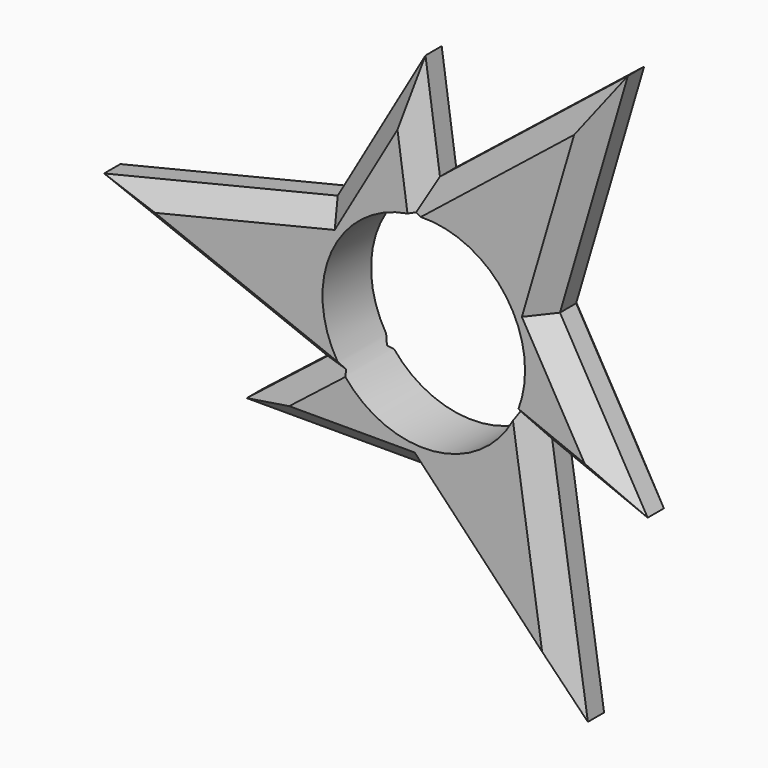
from build123d import *

# Parameters (mm, degrees)
F0_R          = 15
F1_DEPTH      = 9
F2_DEPTH      = 9
F3_T4_DEPTH   = 41.4194656766
F3_T9_DEPTH   = 51.0233182668
F3_T14_DEPTH  = 51.0233182668
F3_T19_DEPTH  = 30.6843352159
F3_T24_DEPTH  = 41.4194656766
F3_T29_DEPTH  = 51.0233182668
F3_T34_DEPTH  = 51.0233182668
F3_T39_DEPTH  = 30.6843352159
F3_T44_DEPTH  = 41.4194656766
F3_T49_DEPTH  = 51.0233182668
F3_T54_DEPTH  = 51.0233182668
F3_T59_DEPTH  = 30.6843352159
F3_T64_DEPTH  = 51.0233182668
F3_T69_DEPTH  = 41.4194656766
F3_T74_DEPTH  = 51.0233182668
F3_T79_DEPTH  = 51.0233182668
F3_T84_DEPTH  = 41.4194656766
F3_T89_DEPTH  = 30.6843352159
F3_T94_DEPTH  = 51.0233182668
F3_T99_DEPTH  = 51.0233182668
F3_T104_DEPTH = 41.4194656766
F3_T109_DEPTH = 51.0233182668
F3_T114_DEPTH = 30.6843352159
F3_T119_DEPTH = 30.6843352159
F3_T125_DEPTH = 51.0233182668
F3_T129_DEPTH = 41.4194656766
F3_T136_DEPTH = 51.0233182668
F3_T140_DEPTH = 30.6843352159
F3_T147_DEPTH = 41.4194656766
F3_T151_DEPTH = 51.0233182668
F3_T158_DEPTH = 51.0233182668
F3_T162_DEPTH = 30.6843352159
F3_T169_DEPTH = 41.4194656766
F3_T173_DEPTH = 51.0233182668
F3_T180_DEPTH = 51.0233182668
F3_T184_DEPTH = 30.6843352159
F3_T191_DEPTH = 41.4194656766
F3_T195_DEPTH = 51.0233182668
F3_T202_DEPTH = 51.0233182668
F3_T206_DEPTH = 30.6843352159
F3_T213_DEPTH = 41.4194656766
F3_T217_DEPTH = 51.0233182668
F3_T224_DEPTH = 51.0233182668
F3_T228_DEPTH = 30.6843352159
F3_T235_DEPTH = 51.0233182668
F3_T239_DEPTH = 41.4194656766
F3_T246_DEPTH = 51.0233182668
F3_T250_DEPTH = 30.6843352159


# Not quite as in the source:
# - a fillet or chamfer that OpenCascade refuses, or shapes differently, is made with other operations: its cross-section is extruded or revolved along the edge and cut away or added


with BuildPart() as f1:
    # F0 (on Front) → F1 (new body)
    with BuildSketch(Plane.XZ):
        with BuildLine():
            ThreePointArc((-16.6111198958, -9.5904345434), (-19.1355906319, 1.3171598584), (-15.1404052923, 11.7759868593))
            Line((-15.1404052923, 11.7759868593), (-49.7397878859, 3.4237381657))
            Line((-49.7397878859, 3.4237381657), (-16.6111198958, -9.5904345434))
        make_face()
        with BuildLine():
            ThreePointArc((0, 19.1808690868), (10.7084892142, 15.9133276745), (17.7685064209, 7.2239821771))
            Line((17.7685064209, 7.2239821771), (27.8349381703, 41.3640508052))
            Line((27.8349381703, 41.3640508052), (0, 19.1808690868))
        make_face()
        with BuildLine():
            Line((21.9048497156, -44.7877889709), (16.6111198958, -9.5904345434))
            ThreePointArc((16.6111198958, -9.5904345434), (8.4271014177, -17.2304875329), (-2.6281011286, -18.9999690364))
            Line((-2.6281011286, -18.9999690364), (21.9048497156, -44.7877889709))
        make_face()
        with BuildLine():
            ThreePointArc((16.6111198958, -9.5904345434), (18.5272968216, -4.9643742213), (19.1808690868, 0))
            ThreePointArc((19.1808690868, 0), (18.8244672495, 3.6803765702), (17.7685064209, 7.2239821771))
            ThreePointArc((17.7685064209, 7.2239821771), (10.7084892142, 15.9133276745), (0, 19.1808690868))
            ThreePointArc((0, 19.1808690868), (-8.4271014177, 17.2304875329), (-15.1404052923, 11.7759868593))
            ThreePointArc((-15.1404052923, 11.7759868593), (-19.1355906319, 1.3171598584), (-16.6111198958, -9.5904345434))
            ThreePointArc((-16.6111198958, -9.5904345434), (-10.7084892142, -15.9133276745), (-2.6281011286, -18.9999690364))
            ThreePointArc((-2.6281011286, -18.9999690364), (8.4271014177, -17.2304875329), (16.6111198958, -9.5904345434))
        make_face()
        Circle(F0_R, mode=Mode.SUBTRACT)
    extrude(amount=F1_DEPTH)

    # F0 (on Front) → F2 (join)
    with BuildSketch(Plane.XZ):
        with BuildLine():
            ThreePointArc((16.6111198958, -9.5904345434), (18.5272968216, -4.9643742213), (19.1808690868, 0))
            ThreePointArc((19.1808690868, 0), (18.8244672495, 3.6803765702), (17.7685064209, 7.2239821771))
            ThreePointArc((17.7685064209, 7.2239821771), (10.7084892142, 15.9133276745), (0, 19.1808690868))
            ThreePointArc((0, 19.1808690868), (-8.4271014177, 17.2304875329), (-15.1404052923, 11.7759868593))
            ThreePointArc((-15.1404052923, 11.7759868593), (-19.1355906319, 1.3171598584), (-16.6111198958, -9.5904345434))
            ThreePointArc((-16.6111198958, -9.5904345434), (-10.7084892142, -15.9133276745), (-2.6281011286, -18.9999690364))
            ThreePointArc((-2.6281011286, -18.9999690364), (8.4271014177, -17.2304875329), (16.6111198958, -9.5904345434))
        make_face()
        Circle(F0_R, mode=Mode.SUBTRACT)
        with BuildLine():
            ThreePointArc((17.7685064209, 7.2239821771), (18.8244672495, 3.6803765702), (19.1808690868, 0))
            ThreePointArc((19.1808690868, 0), (18.5272968216, -4.9643742213), (16.6111198958, -9.5904345434))
            Line((16.6111198958, -9.5904345434), (30.7631902953, -15.2834705217))
            Line((30.7631902953, -15.2834705217), (17.7685064209, 7.2239821771))
        make_face()
        with BuildLine():
            ThreePointArc((0, 19.1808690868), (10.7084892142, 15.9133276745), (17.7685064209, 7.2239821771))
            Line((17.7685064209, 7.2239821771), (27.8349381703, 41.3640508052))
            Line((27.8349381703, 41.3640508052), (0, 19.1808690868))
        make_face()
        with BuildLine():
            Line((21.9048497156, -44.7877889709), (16.6111198958, -9.5904345434))
            ThreePointArc((16.6111198958, -9.5904345434), (8.4271014177, -17.2304875329), (-2.6281011286, -18.9999690364))
            Line((-2.6281011286, -18.9999690364), (21.9048497156, -44.7877889709))
        make_face()
        with BuildLine():
            ThreePointArc((-15.1404052923, 11.7759868593), (-8.4271014177, 17.2304875329), (0, 19.1808690868))
            Line((0, 19.1808690868), (-2.1457214179, 34.2834395581))
            Line((-2.1457214179, 34.2834395581), (-15.1404052923, 11.7759868593))
        make_face()
        with BuildLine():
            Line((-28.6174688775, -18.9999690364), (-2.6281011286, -18.9999690364))
            ThreePointArc((-2.6281011286, -18.9999690364), (-10.7084892142, -15.9133276745), (-16.6111198958, -9.5904345434))
            Line((-16.6111198958, -9.5904345434), (-28.6174688775, -18.9999690364))
        make_face()
        with BuildLine():
            ThreePointArc((-16.6111198958, -9.5904345434), (-19.1355906319, 1.3171598584), (-15.1404052923, 11.7759868593))
            Line((-15.1404052923, 11.7759868593), (-49.7397878859, 3.4237381657))
            Line((-49.7397878859, 3.4237381657), (-16.6111198958, -9.5904345434))
        make_face()
    extrude(amount=F2_DEPTH)

    # F3: chamfer of 3 on 24 edges, made by hand


with BuildPart() as f3_tool2:
    # F3_s3 → F3_t4 (new body)
    with BuildSketch(Plane(origin=(18.1662589207, 0, 31.4648834341), x_dir=(0, 1, 0), z_dir=(-0.5, 0, -0.8660254038))):
        Polygon((-6, -18.9999690364), (-9, -15.9999690364), (-9, -18.9999690364), align=None)
    extrude(amount=F3_T4_DEPTH)

    split(bisect_by=Plane(origin=(-3.5198762352, 0, 14.5811683787), x_dir=(0, 1, 0), z_dir=(-0.2346584157, 0, 0.9720778919)), keep=Keep.TOP)


with BuildPart() as f1_1:
    add(f1.part)

    # F3_t1: cut F3_tool2
    add(f3_tool2.part, mode=Mode.SUBTRACT)


with BuildPart() as f3_tool7:
    # F3_s8 → F3_t9 (new body)
    with BuildSketch(Plane(origin=(-4.1209005243, 0, -0.9947803527), x_dir=(0, 1, 0), z_dir=(-0.9720778919, 0, -0.2346584157))):
        Polygon((-6, -15), (-9, -12), (-9, -15), align=None)
    extrude(amount=F3_T9_DEPTH)

    split(bisect_by=Plane(origin=(-16.4544558566, 0, 9.4999845182), x_dir=(0, 1, 0), z_dir=(-0.8660254038, 0, 0.5)), keep=Keep.TOP)


with BuildPart() as f1_2:
    add(f1_1.part)

    # F3_t6: cut F3_tool7
    add(f3_tool7.part, mode=Mode.SUBTRACT)


with BuildPart() as f3_tool12:
    # F3_s13 → F3_t14 (new body)
    with BuildSketch(Plane(origin=(-51.4360857888, 0, 20.2060072), x_dir=(0, 1, 0), z_dir=(0.930757815, 0, -0.3656362809))):
        Polygon((-6, -15), (-9, -12), (-9, -15), align=None)
    extrude(amount=F3_T14_DEPTH)

    split(bisect_by=Plane(origin=(-1.6642890677, 0, 2.1235944635), x_dir=(0, 1, 0), z_dir=(-0.6168472612, 0, 0.7870828777)), keep=Keep.TOP)


with BuildPart() as f1_3:
    add(f1_2.part)

    # F3_t11: cut F3_tool12
    add(f3_tool12.part, mode=Mode.SUBTRACT)


with BuildPart() as f3_tool17:
    # F3_s18 → F3_t19 (new body)
    with BuildSketch(Plane(origin=(-8.8744478881, 0, -6.9550221835), x_dir=(0, 1, 0), z_dir=(-0.7870828777, 0, -0.6168472612))):
        Polygon((-9, 0.3019430054), (-6, -2.6980569946), (-9, -2.6980569946), align=None)
    extrude(amount=F3_T19_DEPTH)

    split(bisect_by=Plane(origin=(-5.4845442131, 0, -13.9613672244), x_dir=(0, 1, 0), z_dir=(-0.3656362809, 0, -0.930757815)), keep=Keep.TOP)


with BuildPart() as f1_4:
    add(f1_3.part)

    # F3_t16: cut F3_tool17
    add(f3_tool17.part, mode=Mode.SUBTRACT)


with BuildPart() as f3_tool22:
    # F3_s23 → F3_t24 (new body)
    with BuildSketch(Plane.YZ.offset(-36.3325178414)):
        Polygon((-9, -15.9999690364), (-6, -18.9999690364), (-9, -18.9999690364), align=None)
    extrude(amount=F3_T24_DEPTH)

    split(bisect_by=Plane(origin=(-10.8677241153, 0, -10.3388864272), x_dir=(0, 1, 0), z_dir=(-0.724514941, 0, -0.6892590951)), keep=Keep.TOP)


with BuildPart() as f1_5:
    add(f1_4.part)

    # F3_t21: cut F3_tool22
    add(f3_tool22.part, mode=Mode.SUBTRACT)


with BuildPart() as f3_tool27:
    # F3_s28 → F3_t29 (new body)
    with BuildSketch(Plane(origin=(2.9219553188, 0, -3.0714143641), x_dir=(0, 1, 0), z_dir=(0.6892590951, 0, -0.724514941))):
        Polygon((-9, -12), (-6, -15), (-9, -15), align=None)
    extrude(amount=F3_T29_DEPTH)

    split(bisect_by=Plane.XY.offset(-18.9999690364), keep=Keep.BOTTOM)


with BuildPart() as f1_6:
    add(f1_5.part)

    # F3_t26: cut F3_tool27
    add(f3_tool27.part, mode=Mode.SUBTRACT)


with BuildPart() as f3_tool32:
    # F3_s33 → F3_t34 (new body)
    with BuildSketch(Plane(origin=(8.2191273501, 0, -54.6479605643), x_dir=(0, 1, 0), z_dir=(-0.1487285997, 0, 0.988878053))):
        Polygon((-9, -12), (-6, -15), (-9, -15), align=None)
    extrude(amount=F3_T34_DEPTH)

    split(bisect_by=Plane(origin=(-1.0069422189, 0, -2.5031138436), x_dir=(0, 1, 0), z_dir=(-0.3732101364, 0, -0.9277468373)), keep=Keep.TOP)


with BuildPart() as f1_7:
    add(f1_6.part)

    # F3_t31: cut F3_tool32
    add(f3_tool32.part, mode=Mode.SUBTRACT)


with BuildPart() as f3_tool37:
    # F3_s38 → F3_t39 (new body)
    with BuildSketch(Plane(origin=(10.4604498388, 0, -4.207986224), x_dir=(0, 1, 0), z_dir=(0.9277468373, 0, -0.3732101364))):
        Polygon((-9, 0.3019430054), (-6, -2.6980569946), (-9, -2.6980569946), align=None)
    extrude(amount=F3_T39_DEPTH)

    split(bisect_by=Plane(origin=(14.8331707944, 0, 2.2309289955), x_dir=(0, 1, 0), z_dir=(0.988878053, 0, 0.1487285997)), keep=Keep.TOP)


with BuildPart() as f1_8:
    add(f1_7.part)

    # F3_t36: cut F3_tool37
    add(f3_tool37.part, mode=Mode.SUBTRACT)


with BuildPart() as f3_tool42:
    # F3_s43 → F3_t44 (new body)
    with BuildSketch(Plane(origin=(18.1662589207, 0, -31.4648834341), x_dir=(0, 1, 0), z_dir=(-0.5, 0, 0.8660254038))):
        Polygon((-9, -15.9999690364), (-6, -18.9999690364), (-9, -18.9999690364), align=None)
    extrude(amount=F3_T44_DEPTH)

    split(bisect_by=Plane(origin=(14.3876003504, 0, -4.2422819515), x_dir=(0, 1, 0), z_dir=(0.9591733567, 0, -0.2828187968)), keep=Keep.TOP)


with BuildPart() as f1_9:
    add(f1_8.part)

    # F3_t41: cut F3_tool42
    add(f3_tool42.part, mode=Mode.SUBTRACT)


with BuildPart() as f3_tool47:
    # F3_s48 → F3_t49 (new body)
    with BuildSketch(Plane(origin=(1.1989452055, 0, 4.0661947169), x_dir=(0, 1, 0), z_dir=(0.2828187968, 0, 0.9591733567))):
        Polygon((-9, -12), (-6, -15), (-9, -15), align=None)
    extrude(amount=F3_T49_DEPTH)

    split(bisect_by=Plane(origin=(16.4544558566, 0, 9.4999845182), x_dir=(0, 1, 0), z_dir=(0.8660254038, 0, 0.5)), keep=Keep.TOP)


with BuildPart() as f1_10:
    add(f1_9.part)

    # F3_t46: cut F3_tool47
    add(f3_tool47.part, mode=Mode.SUBTRACT)


with BuildPart() as f3_tool52:
    # F3_s53 → F3_t54 (new body)
    with BuildSketch(Plane(origin=(43.2169584386, 0, 34.4419533643), x_dir=(0, 1, 0), z_dir=(-0.7820292153, 0, -0.6232417721))):
        Polygon((-9, -12), (-6, -15), (-9, -15), align=None)
    extrude(amount=F3_T54_DEPTH)

    split(bisect_by=Plane(origin=(2.6712312866, 0, 0.3795193801), x_dir=(0, 1, 0), z_dir=(0.9900573976, 0, 0.1406639596)), keep=Keep.TOP)


with BuildPart() as f1_11:
    add(f1_10.part)

    # F3_t51: cut F3_tool52
    add(f3_tool52.part, mode=Mode.SUBTRACT)


with BuildPart() as f3_tool57:
    # F3_s58 → F3_t59 (new body)
    with BuildSketch(Plane(origin=(-1.5860019507, 0, 11.1630084074), x_dir=(0, 1, 0), z_dir=(-0.1406639596, 0, 0.9900573976))):
        Polygon((-9, 0.3019430054), (-6, -2.6980569946), (-9, -2.6980569946), align=None)
    extrude(amount=F3_T59_DEPTH)

    split(bisect_by=Plane(origin=(-9.3486265813, 0, 11.7304382289), x_dir=(0, 1, 0), z_dir=(-0.6232417721, 0, 0.7820292153)), keep=Keep.TOP)


with BuildPart() as f1_12:
    add(f1_11.part)

    # F3_t56: cut F3_tool57
    add(f3_tool57.part, mode=Mode.SUBTRACT)


with BuildPart() as f3_tool62:
    # F3_s63 → F3_t64 (new body)
    with BuildSketch(Plane(origin=(1.1989452055, 0, 4.0661947169), x_dir=(0, 1, 0), z_dir=(0.2828187968, 0, 0.9591733567))):
        Polygon((0, -12), (-3, -15), (0, -15), align=None)
    extrude(amount=F3_T64_DEPTH)

    split(bisect_by=Plane(origin=(16.4544558566, 0, 9.4999845182), x_dir=(0, 1, 0), z_dir=(0.8660254038, 0, 0.5)), keep=Keep.TOP)


with BuildPart() as f1_13:
    add(f1_12.part)

    # F3_t61: cut F3_tool62
    add(f3_tool62.part, mode=Mode.SUBTRACT)


with BuildPart() as f3_tool67:
    # F3_s68 → F3_t69 (new body)
    with BuildSketch(Plane(origin=(18.1662589207, 0, -31.4648834341), x_dir=(0, 1, 0), z_dir=(-0.5, 0, 0.8660254038))):
        Polygon((0, -15.9999690364), (-3, -18.9999690364), (0, -18.9999690364), align=None)
    extrude(amount=F3_T69_DEPTH)

    split(bisect_by=Plane(origin=(14.3876003504, 0, -4.2422819515), x_dir=(0, 1, 0), z_dir=(0.9591733567, 0, -0.2828187968)), keep=Keep.TOP)


with BuildPart() as f1_14:
    add(f1_13.part)

    # F3_t66: cut F3_tool67
    add(f3_tool67.part, mode=Mode.SUBTRACT)


with BuildPart() as f3_tool72:
    # F3_s73 → F3_t74 (new body)
    with BuildSketch(Plane(origin=(8.2191273501, 0, -54.6479605643), x_dir=(0, 1, 0), z_dir=(-0.1487285997, 0, 0.988878053))):
        Polygon((0, -12), (-3, -15), (0, -15), align=None)
    extrude(amount=F3_T74_DEPTH)

    split(bisect_by=Plane(origin=(-1.0069422189, 0, -2.5031138436), x_dir=(0, 1, 0), z_dir=(-0.3732101364, 0, -0.9277468373)), keep=Keep.TOP)


with BuildPart() as f1_15:
    add(f1_14.part)

    # F3_t71: cut F3_tool72
    add(f3_tool72.part, mode=Mode.SUBTRACT)


with BuildPart() as f3_tool77:
    # F3_s78 → F3_t79 (new body)
    with BuildSketch(Plane(origin=(2.9219553188, 0, -3.0714143641), x_dir=(0, 1, 0), z_dir=(0.6892590951, 0, -0.724514941))):
        Polygon((0, -12), (-3, -15), (0, -15), align=None)
    extrude(amount=F3_T79_DEPTH)

    split(bisect_by=Plane.XY.offset(-18.9999690364), keep=Keep.BOTTOM)


with BuildPart() as f1_16:
    add(f1_15.part)

    # F3_t76: cut F3_tool77
    add(f3_tool77.part, mode=Mode.SUBTRACT)


with BuildPart() as f3_tool82:
    # F3_s83 → F3_t84 (new body)
    with BuildSketch(Plane.YZ.offset(-36.3325178414)):
        Polygon((0, -15.9999690364), (-3, -18.9999690364), (0, -18.9999690364), align=None)
    extrude(amount=F3_T84_DEPTH)

    split(bisect_by=Plane(origin=(-10.8677241153, 0, -10.3388864272), x_dir=(0, 1, 0), z_dir=(-0.724514941, 0, -0.6892590951)), keep=Keep.TOP)


with BuildPart() as f1_17:
    add(f1_16.part)

    # F3_t81: cut F3_tool82
    add(f3_tool82.part, mode=Mode.SUBTRACT)


with BuildPart() as f3_tool87:
    # F3_s88 → F3_t89 (new body)
    with BuildSketch(Plane(origin=(-8.8744478881, 0, -6.9550221835), x_dir=(0, 1, 0), z_dir=(-0.7870828777, 0, -0.6168472612))):
        Polygon((0, 0.3019430054), (-3, -2.6980569946), (0, -2.6980569946), align=None)
    extrude(amount=F3_T89_DEPTH)

    split(bisect_by=Plane(origin=(-5.4845442131, 0, -13.9613672244), x_dir=(0, 1, 0), z_dir=(-0.3656362809, 0, -0.930757815)), keep=Keep.TOP)


with BuildPart() as f1_18:
    add(f1_17.part)

    # F3_t86: cut F3_tool87
    add(f3_tool87.part, mode=Mode.SUBTRACT)


with BuildPart() as f3_tool92:
    # F3_s93 → F3_t94 (new body)
    with BuildSketch(Plane(origin=(-51.4360857888, 0, 20.2060072), x_dir=(0, 1, 0), z_dir=(0.930757815, 0, -0.3656362809))):
        Polygon((-3, -15), (0, -12), (0, -15), align=None)
    extrude(amount=F3_T94_DEPTH)

    split(bisect_by=Plane(origin=(-1.6642890677, 0, 2.1235944635), x_dir=(0, 1, 0), z_dir=(-0.6168472612, 0, 0.7870828777)), keep=Keep.TOP)


with BuildPart() as f1_19:
    add(f1_18.part)

    # F3_t91: cut F3_tool92
    add(f3_tool92.part, mode=Mode.SUBTRACT)


with BuildPart() as f3_tool97:
    # F3_s98 → F3_t99 (new body)
    with BuildSketch(Plane(origin=(-4.1209005243, 0, -0.9947803527), x_dir=(0, 1, 0), z_dir=(-0.9720778919, 0, -0.2346584157))):
        Polygon((-3, -15), (0, -12), (0, -15), align=None)
    extrude(amount=F3_T99_DEPTH)

    split(bisect_by=Plane(origin=(-16.4544558566, 0, 9.4999845182), x_dir=(0, 1, 0), z_dir=(-0.8660254038, 0, 0.5)), keep=Keep.TOP)


with BuildPart() as f1_20:
    add(f1_19.part)

    # F3_t96: cut F3_tool97
    add(f3_tool97.part, mode=Mode.SUBTRACT)


with BuildPart() as f3_tool102:
    # F3_s103 → F3_t104 (new body)
    with BuildSketch(Plane(origin=(18.1662589207, 0, 31.4648834341), x_dir=(0, 1, 0), z_dir=(-0.5, 0, -0.8660254038))):
        Polygon((-3, -18.9999690364), (0, -15.9999690364), (0, -18.9999690364), align=None)
    extrude(amount=F3_T104_DEPTH)

    split(bisect_by=Plane(origin=(-3.5198762352, 0, 14.5811683787), x_dir=(0, 1, 0), z_dir=(-0.2346584157, 0, 0.9720778919)), keep=Keep.TOP)


with BuildPart() as f1_21:
    add(f1_20.part)

    # F3_t101: cut F3_tool102
    add(f3_tool102.part, mode=Mode.SUBTRACT)


with BuildPart() as f3_tool107:
    # F3_s108 → F3_t109 (new body)
    with BuildSketch(Plane(origin=(43.2169584386, 0, 34.4419533643), x_dir=(0, 1, 0), z_dir=(-0.7820292153, 0, -0.6232417721))):
        Polygon((0, -12), (-3, -15), (0, -15), align=None)
    extrude(amount=F3_T109_DEPTH)

    split(bisect_by=Plane(origin=(2.6712312866, 0, 0.3795193801), x_dir=(0, 1, 0), z_dir=(0.9900573976, 0, 0.1406639596)), keep=Keep.TOP)


with BuildPart() as f1_22:
    add(f1_21.part)

    # F3_t106: cut F3_tool107
    add(f3_tool107.part, mode=Mode.SUBTRACT)


with BuildPart() as f3_tool112:
    # F3_s113 → F3_t114 (new body)
    with BuildSketch(Plane(origin=(10.4604498388, 0, -4.207986224), x_dir=(0, 1, 0), z_dir=(0.9277468373, 0, -0.3732101364))):
        Polygon((0, 0.3019430054), (-3, -2.6980569946), (0, -2.6980569946), align=None)
    extrude(amount=F3_T114_DEPTH)

    split(bisect_by=Plane(origin=(14.8331707944, 0, 2.2309289955), x_dir=(0, 1, 0), z_dir=(0.988878053, 0, 0.1487285997)), keep=Keep.TOP)


with BuildPart() as f1_23:
    add(f1_22.part)

    # F3_t111: cut F3_tool112
    add(f3_tool112.part, mode=Mode.SUBTRACT)


with BuildPart() as f3_tool117:
    # F3_s118 → F3_t119 (new body)
    with BuildSketch(Plane(origin=(-1.5860019507, 0, 11.1630084074), x_dir=(0, 1, 0), z_dir=(-0.1406639596, 0, 0.9900573976))):
        Polygon((0, 0.3019430054), (-3, -2.6980569946), (0, -2.6980569946), align=None)
    extrude(amount=F3_T119_DEPTH)

    split(bisect_by=Plane(origin=(-9.3486265813, 0, 11.7304382289), x_dir=(0, 1, 0), z_dir=(-0.6232417721, 0, 0.7820292153)), keep=Keep.TOP)


with BuildPart() as f1_24:
    add(f1_23.part)

    # F3_t116: cut F3_tool117
    add(f3_tool117.part, mode=Mode.SUBTRACT)


with BuildPart() as f3_tool123:
    # F3_s124 → F3_t125 (new body)
    with BuildSketch(Plane(origin=(-4.1209005243, 0, -0.9947803527), x_dir=(0, 1, 0), z_dir=(-0.9720778919, 0, -0.2346584157))):
        Polygon((-6, -15), (-9, -12), (-9, -15), align=None)
    extrude(amount=F3_T125_DEPTH)

    split(bisect_by=Plane(origin=(-16.4544558566, 0, 9.4999845182), x_dir=(0, 1, 0), z_dir=(0.8660254038, 0, -0.5)), keep=Keep.TOP)


with BuildPart() as f3_tool127:
    # F3_s128 → F3_t129 (new body)
    with BuildSketch(Plane(origin=(18.1662589207, 0, 31.4648834341), x_dir=(0, 1, 0), z_dir=(-0.5, 0, -0.8660254038))):
        Polygon((-6, -18.9999690364), (-9, -15.9999690364), (-9, -18.9999690364), align=None)
    extrude(amount=F3_T129_DEPTH)

    split(bisect_by=Plane(origin=(-3.5198762352, 0, 14.5811683787), x_dir=(0, 1, 0), z_dir=(0.2346584157, 0, -0.9720778919)), keep=Keep.TOP)


with BuildPart() as f3_tool123_1:
    add(f3_tool123.part)

    # F3_t131: intersect F3_tool127
    add(f3_tool127.part, mode=Mode.INTERSECT)


with BuildPart() as f1_25:
    add(f1_24.part)

    # F3_t121: cut F3_tool123
    add(f3_tool123_1.part, mode=Mode.SUBTRACT)


with BuildPart() as f3_tool134:
    # F3_s135 → F3_t136 (new body)
    with BuildSketch(Plane(origin=(-51.4360857888, 0, 20.2060072), x_dir=(0, 1, 0), z_dir=(0.930757815, 0, -0.3656362809))):
        Polygon((-6, -15), (-9, -12), (-9, -15), align=None)
    extrude(amount=F3_T136_DEPTH)

    split(bisect_by=Plane(origin=(-1.6642890677, 0, 2.1235944635), x_dir=(0, 1, 0), z_dir=(0.6168472612, 0, -0.7870828777)), keep=Keep.TOP)


with BuildPart() as f3_tool138:
    # F3_s139 → F3_t140 (new body)
    with BuildSketch(Plane(origin=(-8.8744478881, 0, -6.9550221835), x_dir=(0, 1, 0), z_dir=(-0.7870828777, 0, -0.6168472612))):
        Polygon((-9, 0.3019430054), (-6, -2.6980569946), (-9, -2.6980569946), align=None)
    extrude(amount=F3_T140_DEPTH)

    split(bisect_by=Plane(origin=(-5.4845442131, 0, -13.9613672244), x_dir=(0, 1, 0), z_dir=(0.3656362809, 0, 0.930757815)), keep=Keep.TOP)


with BuildPart() as f3_tool134_1:
    add(f3_tool134.part)

    # F3_t142: intersect F3_tool138
    add(f3_tool138.part, mode=Mode.INTERSECT)


with BuildPart() as f1_26:
    add(f1_25.part)

    # F3_t132: cut F3_tool134
    add(f3_tool134_1.part, mode=Mode.SUBTRACT)


with BuildPart() as f3_tool145:
    # F3_s146 → F3_t147 (new body)
    with BuildSketch(Plane.YZ.offset(-36.3325178414)):
        Polygon((-9, -15.9999690364), (-6, -18.9999690364), (-9, -18.9999690364), align=None)
    extrude(amount=F3_T147_DEPTH)

    split(bisect_by=Plane(origin=(-10.8677241153, 0, -10.3388864272), x_dir=(0, 1, 0), z_dir=(0.724514941, 0, 0.6892590951)), keep=Keep.TOP)


with BuildPart() as f3_tool149:
    # F3_s150 → F3_t151 (new body)
    with BuildSketch(Plane(origin=(2.9219553188, 0, -3.0714143641), x_dir=(0, 1, 0), z_dir=(0.6892590951, 0, -0.724514941))):
        Polygon((-9, -12), (-6, -15), (-9, -15), align=None)
    extrude(amount=F3_T151_DEPTH)

    split(bisect_by=Plane.XY.offset(-18.9999690364), keep=Keep.TOP)


with BuildPart() as f3_tool145_1:
    add(f3_tool145.part)

    # F3_t153: intersect F3_tool149
    add(f3_tool149.part, mode=Mode.INTERSECT)


with BuildPart() as f1_27:
    add(f1_26.part)

    # F3_t143: cut F3_tool145
    add(f3_tool145_1.part, mode=Mode.SUBTRACT)


with BuildPart() as f3_tool156:
    # F3_s157 → F3_t158 (new body)
    with BuildSketch(Plane(origin=(8.2191273501, 0, -54.6479605643), x_dir=(0, 1, 0), z_dir=(-0.1487285997, 0, 0.988878053))):
        Polygon((-9, -12), (-6, -15), (-9, -15), align=None)
    extrude(amount=F3_T158_DEPTH)

    split(bisect_by=Plane(origin=(-1.0069422189, 0, -2.5031138436), x_dir=(0, 1, 0), z_dir=(0.3732101364, 0, 0.9277468373)), keep=Keep.TOP)


with BuildPart() as f3_tool160:
    # F3_s161 → F3_t162 (new body)
    with BuildSketch(Plane(origin=(10.4604498388, 0, -4.207986224), x_dir=(0, 1, 0), z_dir=(0.9277468373, 0, -0.3732101364))):
        Polygon((-9, 0.3019430054), (-6, -2.6980569946), (-9, -2.6980569946), align=None)
    extrude(amount=F3_T162_DEPTH)

    split(bisect_by=Plane(origin=(14.8331707944, 0, 2.2309289955), x_dir=(0, 1, 0), z_dir=(-0.988878053, 0, -0.1487285997)), keep=Keep.TOP)


with BuildPart() as f3_tool156_1:
    add(f3_tool156.part)

    # F3_t164: intersect F3_tool160
    add(f3_tool160.part, mode=Mode.INTERSECT)


with BuildPart() as f1_28:
    add(f1_27.part)

    # F3_t154: cut F3_tool156
    add(f3_tool156_1.part, mode=Mode.SUBTRACT)


with BuildPart() as f3_tool167:
    # F3_s168 → F3_t169 (new body)
    with BuildSketch(Plane(origin=(18.1662589207, 0, -31.4648834341), x_dir=(0, 1, 0), z_dir=(-0.5, 0, 0.8660254038))):
        Polygon((-9, -15.9999690364), (-6, -18.9999690364), (-9, -18.9999690364), align=None)
    extrude(amount=F3_T169_DEPTH)

    split(bisect_by=Plane(origin=(14.3876003504, 0, -4.2422819515), x_dir=(0, 1, 0), z_dir=(-0.9591733567, 0, 0.2828187968)), keep=Keep.TOP)


with BuildPart() as f3_tool171:
    # F3_s172 → F3_t173 (new body)
    with BuildSketch(Plane(origin=(1.1989452055, 0, 4.0661947169), x_dir=(0, 1, 0), z_dir=(0.2828187968, 0, 0.9591733567))):
        Polygon((-9, -12), (-6, -15), (-9, -15), align=None)
    extrude(amount=F3_T173_DEPTH)

    split(bisect_by=Plane(origin=(16.4544558566, 0, 9.4999845182), x_dir=(0, 1, 0), z_dir=(-0.8660254038, 0, -0.5)), keep=Keep.TOP)


with BuildPart() as f3_tool167_1:
    add(f3_tool167.part)

    # F3_t175: intersect F3_tool171
    add(f3_tool171.part, mode=Mode.INTERSECT)


with BuildPart() as f1_29:
    add(f1_28.part)

    # F3_t165: cut F3_tool167
    add(f3_tool167_1.part, mode=Mode.SUBTRACT)


with BuildPart() as f3_tool178:
    # F3_s179 → F3_t180 (new body)
    with BuildSketch(Plane(origin=(43.2169584386, 0, 34.4419533643), x_dir=(0, 1, 0), z_dir=(-0.7820292153, 0, -0.6232417721))):
        Polygon((-9, -12), (-6, -15), (-9, -15), align=None)
    extrude(amount=F3_T180_DEPTH)

    split(bisect_by=Plane(origin=(2.6712312866, 0, 0.3795193801), x_dir=(0, 1, 0), z_dir=(-0.9900573976, 0, -0.1406639596)), keep=Keep.TOP)


with BuildPart() as f3_tool182:
    # F3_s183 → F3_t184 (new body)
    with BuildSketch(Plane(origin=(-1.5860019507, 0, 11.1630084074), x_dir=(0, 1, 0), z_dir=(-0.1406639596, 0, 0.9900573976))):
        Polygon((-9, 0.3019430054), (-6, -2.6980569946), (-9, -2.6980569946), align=None)
    extrude(amount=F3_T184_DEPTH)

    split(bisect_by=Plane(origin=(-9.3486265813, 0, 11.7304382289), x_dir=(0, 1, 0), z_dir=(0.6232417721, 0, -0.7820292153)), keep=Keep.TOP)


with BuildPart() as f3_tool178_1:
    add(f3_tool178.part)

    # F3_t186: intersect F3_tool182
    add(f3_tool182.part, mode=Mode.INTERSECT)


with BuildPart() as f1_30:
    add(f1_29.part)

    # F3_t176: cut F3_tool178
    add(f3_tool178_1.part, mode=Mode.SUBTRACT)


with BuildPart() as f3_tool189:
    # F3_s190 → F3_t191 (new body)
    with BuildSketch(Plane(origin=(18.1662589207, 0, -31.4648834341), x_dir=(0, 1, 0), z_dir=(-0.5, 0, 0.8660254038))):
        Polygon((0, -15.9999690364), (-3, -18.9999690364), (0, -18.9999690364), align=None)
    extrude(amount=F3_T191_DEPTH)

    split(bisect_by=Plane(origin=(14.3876003504, 0, -4.2422819515), x_dir=(0, 1, 0), z_dir=(-0.9591733567, 0, 0.2828187968)), keep=Keep.TOP)


with BuildPart() as f3_tool193:
    # F3_s194 → F3_t195 (new body)
    with BuildSketch(Plane(origin=(1.1989452055, 0, 4.0661947169), x_dir=(0, 1, 0), z_dir=(0.2828187968, 0, 0.9591733567))):
        Polygon((0, -12), (-3, -15), (0, -15), align=None)
    extrude(amount=F3_T195_DEPTH)

    split(bisect_by=Plane(origin=(16.4544558566, 0, 9.4999845182), x_dir=(0, 1, 0), z_dir=(-0.8660254038, 0, -0.5)), keep=Keep.TOP)


with BuildPart() as f3_tool189_1:
    add(f3_tool189.part)

    # F3_t197: intersect F3_tool193
    add(f3_tool193.part, mode=Mode.INTERSECT)


with BuildPart() as f1_31:
    add(f1_30.part)

    # F3_t187: cut F3_tool189
    add(f3_tool189_1.part, mode=Mode.SUBTRACT)


with BuildPart() as f3_tool200:
    # F3_s201 → F3_t202 (new body)
    with BuildSketch(Plane(origin=(8.2191273501, 0, -54.6479605643), x_dir=(0, 1, 0), z_dir=(-0.1487285997, 0, 0.988878053))):
        Polygon((0, -12), (-3, -15), (0, -15), align=None)
    extrude(amount=F3_T202_DEPTH)

    split(bisect_by=Plane(origin=(-1.0069422189, 0, -2.5031138436), x_dir=(0, 1, 0), z_dir=(0.3732101364, 0, 0.9277468373)), keep=Keep.TOP)


with BuildPart() as f3_tool204:
    # F3_s205 → F3_t206 (new body)
    with BuildSketch(Plane(origin=(10.4604498388, 0, -4.207986224), x_dir=(0, 1, 0), z_dir=(0.9277468373, 0, -0.3732101364))):
        Polygon((0, 0.3019430054), (-3, -2.6980569946), (0, -2.6980569946), align=None)
    extrude(amount=F3_T206_DEPTH)

    split(bisect_by=Plane(origin=(14.8331707944, 0, 2.2309289955), x_dir=(0, 1, 0), z_dir=(-0.988878053, 0, -0.1487285997)), keep=Keep.TOP)


with BuildPart() as f3_tool200_1:
    add(f3_tool200.part)

    # F3_t208: intersect F3_tool204
    add(f3_tool204.part, mode=Mode.INTERSECT)


with BuildPart() as f1_32:
    add(f1_31.part)

    # F3_t198: cut F3_tool200
    add(f3_tool200_1.part, mode=Mode.SUBTRACT)


with BuildPart() as f3_tool211:
    # F3_s212 → F3_t213 (new body)
    with BuildSketch(Plane.YZ.offset(-36.3325178414)):
        Polygon((0, -15.9999690364), (-3, -18.9999690364), (0, -18.9999690364), align=None)
    extrude(amount=F3_T213_DEPTH)

    split(bisect_by=Plane(origin=(-10.8677241153, 0, -10.3388864272), x_dir=(0, 1, 0), z_dir=(0.724514941, 0, 0.6892590951)), keep=Keep.TOP)


with BuildPart() as f3_tool215:
    # F3_s216 → F3_t217 (new body)
    with BuildSketch(Plane(origin=(2.9219553188, 0, -3.0714143641), x_dir=(0, 1, 0), z_dir=(0.6892590951, 0, -0.724514941))):
        Polygon((0, -12), (-3, -15), (0, -15), align=None)
    extrude(amount=F3_T217_DEPTH)

    split(bisect_by=Plane.XY.offset(-18.9999690364), keep=Keep.TOP)


with BuildPart() as f3_tool211_1:
    add(f3_tool211.part)

    # F3_t219: intersect F3_tool215
    add(f3_tool215.part, mode=Mode.INTERSECT)


with BuildPart() as f1_33:
    add(f1_32.part)

    # F3_t209: cut F3_tool211
    add(f3_tool211_1.part, mode=Mode.SUBTRACT)


with BuildPart() as f3_tool222:
    # F3_s223 → F3_t224 (new body)
    with BuildSketch(Plane(origin=(-51.4360857888, 0, 20.2060072), x_dir=(0, 1, 0), z_dir=(0.930757815, 0, -0.3656362809))):
        Polygon((-3, -15), (0, -12), (0, -15), align=None)
    extrude(amount=F3_T224_DEPTH)

    split(bisect_by=Plane(origin=(-1.6642890677, 0, 2.1235944635), x_dir=(0, 1, 0), z_dir=(0.6168472612, 0, -0.7870828777)), keep=Keep.TOP)


with BuildPart() as f3_tool226:
    # F3_s227 → F3_t228 (new body)
    with BuildSketch(Plane(origin=(-8.8744478881, 0, -6.9550221835), x_dir=(0, 1, 0), z_dir=(-0.7870828777, 0, -0.6168472612))):
        Polygon((0, 0.3019430054), (-3, -2.6980569946), (0, -2.6980569946), align=None)
    extrude(amount=F3_T228_DEPTH)

    split(bisect_by=Plane(origin=(-5.4845442131, 0, -13.9613672244), x_dir=(0, 1, 0), z_dir=(0.3656362809, 0, 0.930757815)), keep=Keep.TOP)


with BuildPart() as f3_tool222_1:
    add(f3_tool222.part)

    # F3_t230: intersect F3_tool226
    add(f3_tool226.part, mode=Mode.INTERSECT)


with BuildPart() as f1_34:
    add(f1_33.part)

    # F3_t220: cut F3_tool222
    add(f3_tool222_1.part, mode=Mode.SUBTRACT)


with BuildPart() as f3_tool233:
    # F3_s234 → F3_t235 (new body)
    with BuildSketch(Plane(origin=(-4.1209005243, 0, -0.9947803527), x_dir=(0, 1, 0), z_dir=(-0.9720778919, 0, -0.2346584157))):
        Polygon((-3, -15), (0, -12), (0, -15), align=None)
    extrude(amount=F3_T235_DEPTH)

    split(bisect_by=Plane(origin=(-16.4544558566, 0, 9.4999845182), x_dir=(0, 1, 0), z_dir=(0.8660254038, 0, -0.5)), keep=Keep.TOP)


with BuildPart() as f3_tool237:
    # F3_s238 → F3_t239 (new body)
    with BuildSketch(Plane(origin=(18.1662589207, 0, 31.4648834341), x_dir=(0, 1, 0), z_dir=(-0.5, 0, -0.8660254038))):
        Polygon((-3, -18.9999690364), (0, -15.9999690364), (0, -18.9999690364), align=None)
    extrude(amount=F3_T239_DEPTH)

    split(bisect_by=Plane(origin=(-3.5198762352, 0, 14.5811683787), x_dir=(0, 1, 0), z_dir=(0.2346584157, 0, -0.9720778919)), keep=Keep.TOP)


with BuildPart() as f3_tool233_1:
    add(f3_tool233.part)

    # F3_t241: intersect F3_tool237
    add(f3_tool237.part, mode=Mode.INTERSECT)


with BuildPart() as f1_35:
    add(f1_34.part)

    # F3_t231: cut F3_tool233
    add(f3_tool233_1.part, mode=Mode.SUBTRACT)


with BuildPart() as f3_tool244:
    # F3_s245 → F3_t246 (new body)
    with BuildSketch(Plane(origin=(43.2169584386, 0, 34.4419533643), x_dir=(0, 1, 0), z_dir=(-0.7820292153, 0, -0.6232417721))):
        Polygon((0, -12), (-3, -15), (0, -15), align=None)
    extrude(amount=F3_T246_DEPTH)

    split(bisect_by=Plane(origin=(2.6712312866, 0, 0.3795193801), x_dir=(0, 1, 0), z_dir=(-0.9900573976, 0, -0.1406639596)), keep=Keep.TOP)


with BuildPart() as f3_tool248:
    # F3_s249 → F3_t250 (new body)
    with BuildSketch(Plane(origin=(-1.5860019507, 0, 11.1630084074), x_dir=(0, 1, 0), z_dir=(-0.1406639596, 0, 0.9900573976))):
        Polygon((0, 0.3019430054), (-3, -2.6980569946), (0, -2.6980569946), align=None)
    extrude(amount=F3_T250_DEPTH)

    split(bisect_by=Plane(origin=(-9.3486265813, 0, 11.7304382289), x_dir=(0, 1, 0), z_dir=(0.6232417721, 0, -0.7820292153)), keep=Keep.TOP)


with BuildPart() as f3_tool244_1:
    add(f3_tool244.part)

    # F3_t252: intersect F3_tool248
    add(f3_tool248.part, mode=Mode.INTERSECT)


with BuildPart() as f1_36:
    add(f1_35.part)

    # F3_t242: cut F3_tool244
    add(f3_tool244_1.part, mode=Mode.SUBTRACT)


solid = f1_36.part
